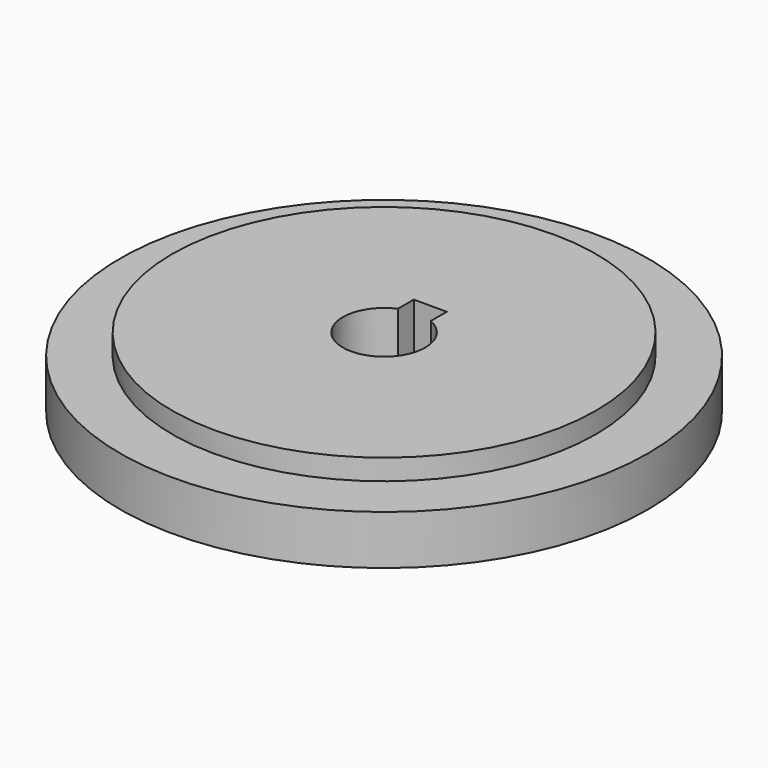
from build123d import *

# Parameters (mm, degrees)
F0_R          = 50.8
F0_R_2        = 7.9375
F1_DEPTH      = 4.5
F1_DEPTH_BACK = 5
F2_R          = 40.8
F2_R_2        = 7.9375
F3_DEPTH      = 4
F4_W          = 6.35
F4_H          = 6.35
F5_DEPTH      = 17.001


# Not quite as in the source:
# - a pattern or mirror of a feature is missing from the dataset's text; its kind, count and spacing are read off the source's solid


with BuildPart() as f1:
    # F0 (on Top) → F1 (new body, two sides)
    with BuildSketch(Plane.XY) as f1_sk:
        Circle(F0_R)
        Circle(F0_R_2, mode=Mode.SUBTRACT)
    extrude(amount=F1_DEPTH)
    extrude(f1_sk.sketch, amount=-F1_DEPTH_BACK)

    # F2 (on face) → F3 (join)
    with BuildSketch(Plane.XY.offset(4.5)):
        Circle(F2_R)
        Circle(F2_R_2, mode=Mode.SUBTRACT)
    f3 = extrude(amount=F3_DEPTH)

    # F3_copies: F3 across plane
    add(f3.mirror(Plane(origin=(0, 0, 0), x_dir=(-1, 0, 0), z_dir=(0, 0, -1))))

    # F4 (on face) → F5 (cut, through all)
    with BuildSketch(Plane.XY.offset(8.5)):
        with Locations((0, 7.9375)):
            Rectangle(F4_W, F4_H)
    extrude(amount=-F5_DEPTH, mode=Mode.SUBTRACT)


solid = f1.part
